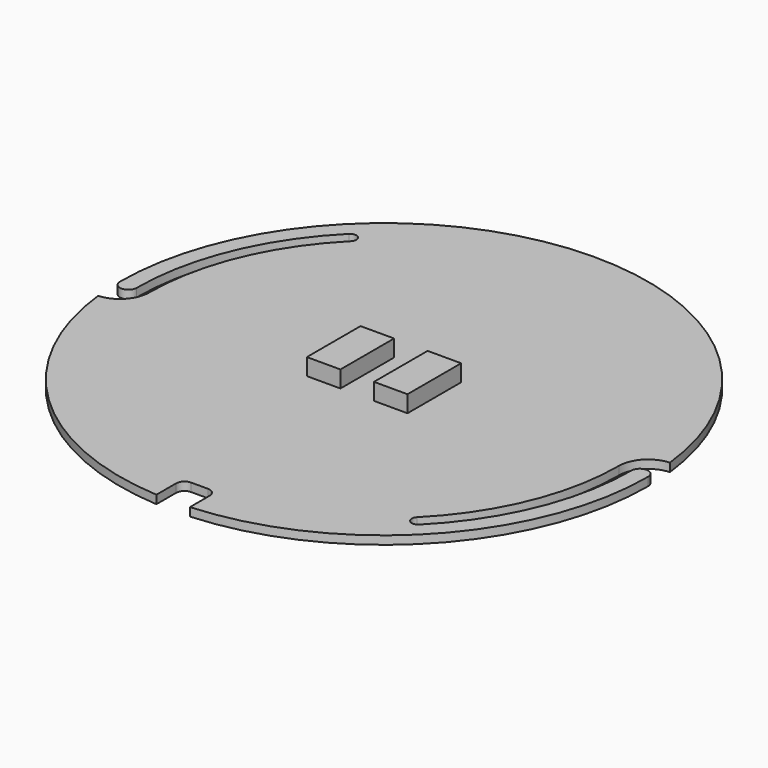
from build123d import *

# Parameters (mm, degrees)
F0_R     = 7.875
F1_DEPTH = 0.25
F2_W     = 1
F2_H     = 2
F3_DEPTH = 0.5
F5_DEPTH = 0.5
F7_DEPTH = 1


# Not quite as in the source:
# - a feature names something its author has since deleted; it is built from what else it names


with BuildPart() as f1:
    # F0 (on Top) → F1 (new body)
    with BuildSketch(Plane.XY):
        Circle(F0_R)
    extrude(amount=F1_DEPTH)

    # F2 (on face) → F3 (join)
    with BuildSketch(Plane.XY.offset(0.25)):
        with Locations((-1, 0)):
            Rectangle(F2_W, F2_H)
        with Locations((1, 0)):
            Rectangle(F2_W, F2_H)
    extrude(amount=F3_DEPTH)

    # F4 (on face) → F5 (cut)
    with BuildSketch(Plane.XY.offset(0.25)):
        with BuildLine():
            ThreePointArc((-0.5, -7.8591109548), (0, -7.875), (0.5, -7.8591109548))
            Line((0.5, -7.8591109548), (0.5, -7.125))
            ThreePointArc((0.5, -7.125), (0.4267766953, -6.9482233047), (0.25, -6.875))
            Line((0.25, -6.875), (-0.25, -6.875))
            ThreePointArc((-0.25, -6.875), (-0.4267766953, -6.9482233047), (-0.5, -7.125))
            Line((-0.5, -7.125), (-0.5, -7.8591109548))
        make_face()
    extrude(amount=-F5_DEPTH, mode=Mode.SUBTRACT)

    # F6 (on face) → F7 (cut)
    with BuildSketch(Plane.XY.offset(0.25)):
        with BuildLine():
            ThreePointArc((-5.2149125113, 5.2149125113), (-6.8136115523, 2.8222903137), (-7.375, 0))
            ThreePointArc((-7.375, 0), (-7.625, -0.25), (-7.875, 0))
            ThreePointArc((-7.875, 0), (-7.8628378306, -0.4375), (-7.8263888889, -0.8736486478))
            ThreePointArc((-7.8263888889, -0.8736486478), (-7.2393272374, -0.6012862371), (-7, 0))
            ThreePointArc((-7, 0), (-6.4671567276, 2.6787840266), (-4.9497474683, 4.9497474683))
            ThreePointArc((-4.9497474683, 4.9497474683), (-4.9497474683, 5.2149125113), (-5.2149125113, 5.2149125113))
        make_face()
        with BuildLine():
            ThreePointArc((7.875, 0), (7.8628378306, 0.4375), (7.8263888889, 0.8736486478))
            ThreePointArc((7.8263888889, 0.8736486478), (7.2393272374, 0.6012862371), (7, 0))
            ThreePointArc((7, 0), (6.4671567276, -2.6787840266), (4.9497474683, -4.9497474683))
            ThreePointArc((4.9497474683, -4.9497474683), (4.9497474683, -5.2149125113), (5.2149125113, -5.2149125113))
            ThreePointArc((5.2149125113, -5.2149125113), (6.8136115523, -2.8222903137), (7.375, 0))
            ThreePointArc((7.375, 0), (7.625, 0.25), (7.875, 0))
        make_face()
    extrude(amount=-F7_DEPTH, mode=Mode.SUBTRACT)


solid = f1.part
